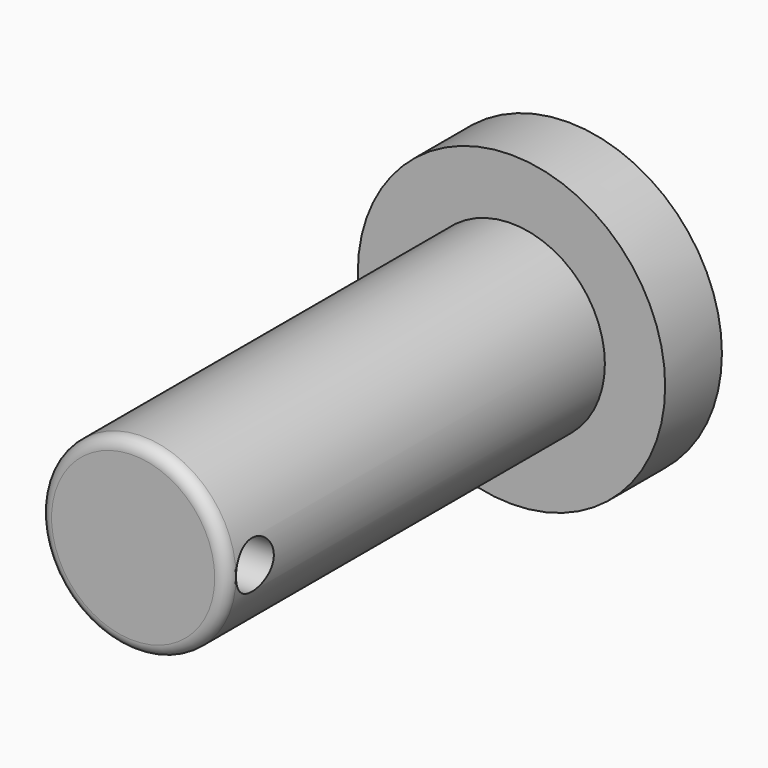
from build123d import *

# Parameters (mm, degrees)
F0_R     = 6.5
F1_DEPTH = 3
F2_R     = 3.95
F3_DEPTH = 20
F5_R     = 1
F6_DEPTH = 10.451
F7_R     = 0.4999


# Not quite as in the source:
# - a fillet or chamfer is up to 0.001 mm smaller than in the source, because OpenCascade refuses the exact size


with BuildPart() as f1:
    # F0 (on Front) → F1 (new body)
    with BuildSketch(Plane.XZ):
        Circle(F0_R)
    extrude(amount=F1_DEPTH)

    # F2 (on face) → F3 (join)
    with BuildSketch(Plane.XZ.offset(3)):
        Circle(F2_R)
    extrude(amount=F3_DEPTH)

    # F5 (on offset) → F6 (cut, through all)
    with BuildSketch(Plane.YZ.offset(3.95)):
        with Locations((-21.5, 0)):
            Circle(F5_R)
    extrude(amount=-F6_DEPTH, mode=Mode.SUBTRACT)

    # F7 (radius 0.5 in the source; OpenCascade refuses exactly that, so slightly less here)
    f7_edges = [f1.edges().sort_by_distance(p)[0] for p in [
        (-3.95, -23, 0),
    ]]
    fillet(f7_edges, radius=F7_R)


with BuildPart() as f8_1:
    # F8: copy of F1
    add(f1.part)


solid = Compound([f1.part, f8_1.part])
